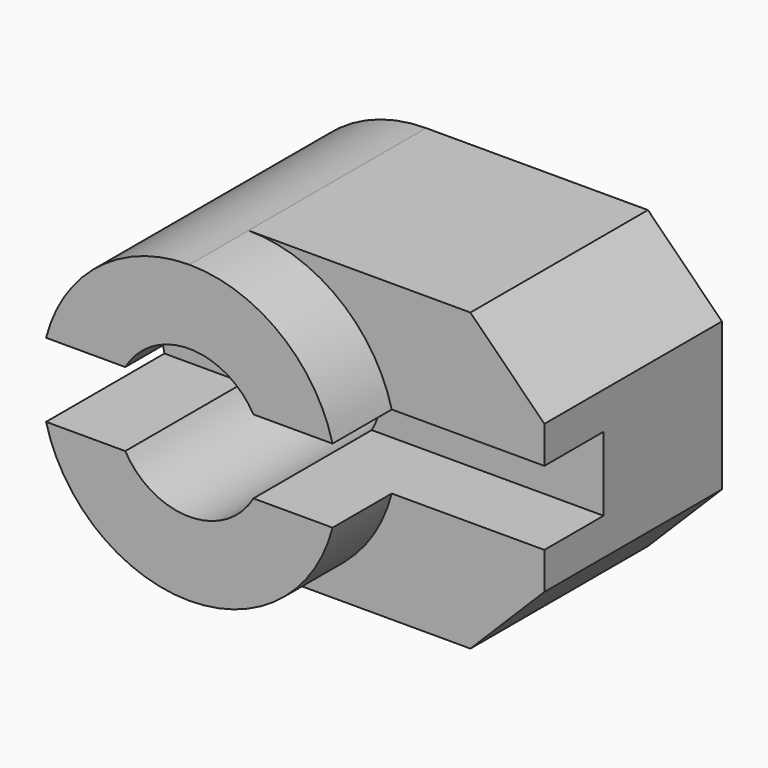
from build123d import *

# Parameters (mm, degrees)
F1_DEPTH = 20
F2_R     = 9.99999
F4_DEPTH = 25
F5_R     = 5
F6_DEPTH = 20.001
F7_R     = 9.99999
F8_W     = 10
F8_H     = 5
F9_DEPTH = 30.001


# Not quite as in the source:
# - a fillet or chamfer is up to 0.001 mm smaller than in the source, because OpenCascade refuses the exact size


with BuildPart() as f1:
    # F0 (on Top) → F1 (new body)
    with BuildSketch(Plane.XY):
        Polygon((30, 20), (0, 20), (0, 0), (20, 0), (20, 5), (30, 5), align=None)
    extrude(amount=F1_DEPTH)

    # F2 (radius 10 in the source; OpenCascade refuses exactly that, so slightly less here)
    f2_edges = [f1.edges().sort_by_distance(p)[0] for p in [
        (0, 10, 20),
        (0, 10, 0),
    ]]
    fillet(f2_edges, radius=F2_R)

    # F3 (on Front) → F4 (cut)
    with BuildSketch(Plane.XZ):
        Polygon((30, 20), (25, 20), (30, 15), align=None)
        Polygon((30, 0), (30, 5), (25, 0), align=None)
    extrude(amount=-F4_DEPTH, mode=Mode.SUBTRACT)

    # F5 (on face) → F6 (cut, through all)
    with BuildSketch(Plane.XZ):
        with Locations((10, 10)):
            Circle(F5_R)
    extrude(amount=-F6_DEPTH, mode=Mode.SUBTRACT)

    # F7 (radius 10 in the source; OpenCascade refuses exactly that, so slightly less here)
    f7_edges = [f1.edges().sort_by_distance(p)[0] for p in [
        (20, 2.5, 20),
        (20, 2.5, 0),
    ]]
    fillet(f7_edges, radius=F7_R)

    # F8 (on Right) → F9 (cut, through all)
    with BuildSketch(Plane.YZ):
        with Locations((5, 10)):
            Rectangle(F8_W, F8_H)
    extrude(amount=F9_DEPTH, mode=Mode.SUBTRACT)


solid = f1.part
